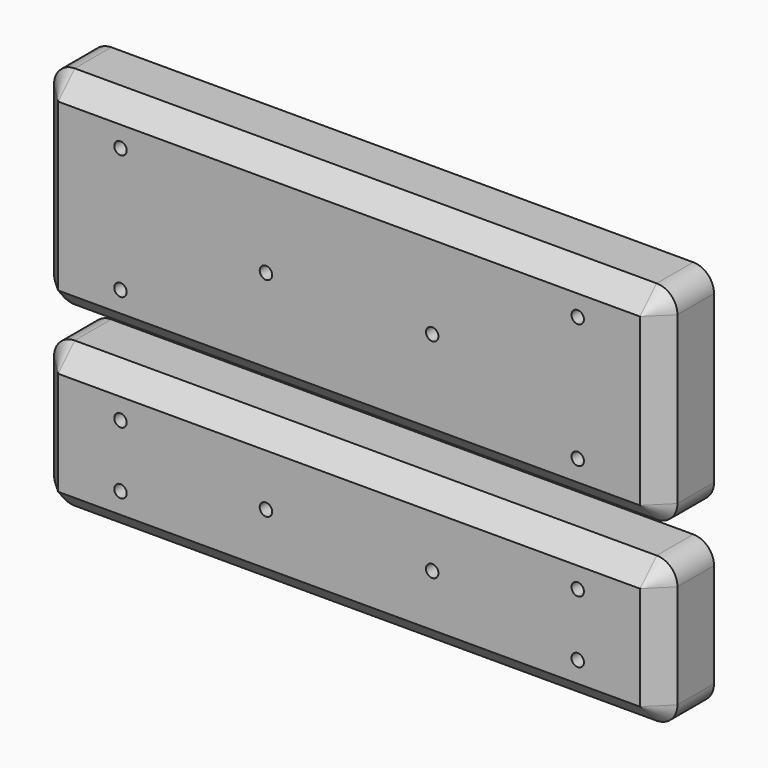
from build123d import *

# Parameters (mm, degrees)
F0_R      = 1.5
F1_DEPTH  = 16
F2_SIZE   = 4.99999
F2_2_SIZE = 4.99999


# Not quite as in the source:
# - a fillet or chamfer is up to 0.001 mm smaller than in the source, because OpenCascade refuses the exact size


with BuildPart() as f1:
    # F0 (on Front) → F1 (new body)
    with BuildSketch(Plane.XZ):
        with BuildLine():
            Line((70, 25), (-70, 25))
            ThreePointArc((-70, 25), (-73.5355339059, 23.5355339059), (-75, 20))
            Line((-75, 20), (-75, -20))
            ThreePointArc((-75, -20), (-73.5355339059, -23.5355339059), (-70, -25))
            Line((-70, -25), (70, -25))
            ThreePointArc((70, -25), (73.5355339059, -23.5355339059), (75, -20))
            Line((75, -20), (75, 20))
            ThreePointArc((75, 20), (73.5355339059, 23.5355339059), (70, 25))
        make_face()
        with Locations((-55, -15)):
            Circle(F0_R, mode=Mode.SUBTRACT)
        with Locations((-20, 0)):
            Circle(F0_R, mode=Mode.SUBTRACT)
        with Locations((-55, 15)):
            Circle(F0_R, mode=Mode.SUBTRACT)
        with Locations((20, 0)):
            Circle(F0_R, mode=Mode.SUBTRACT)
        with Locations((55, -15)):
            Circle(F0_R, mode=Mode.SUBTRACT)
        with Locations((55, 15)):
            Circle(F0_R, mode=Mode.SUBTRACT)
    extrude(amount=F1_DEPTH)

    # F2 (size 5 in the source; OpenCascade refuses exactly that, so slightly less here)
    f2_edges = [f1.edges().sort_by_distance(p)[0] for p in [
        (0, -16, 25),
        (-73.535534, -16, 23.535534),
        (-75, -16, 0),
        (-73.535534, -16, -23.535534),
        (0, -16, -25),
        (73.535534, -16, -23.535534),
        (75, -16, 0),
        (73.535534, -16, 23.535534),
    ]]
    chamfer(f2_edges, length=F2_SIZE)


with BuildPart() as f1b:
    # F0 (on Front) → F1, piece 2 (new body)
    with BuildSketch(Plane.XZ):
        with BuildLine():
            ThreePointArc((-70, -32.6368902624), (-73.5355339059, -34.1013563564), (-75, -37.6368902624))
            Line((-75, -37.6368902624), (-75, -62.6368902624))
            ThreePointArc((-75, -62.6368902624), (-73.5355339059, -66.1724241683), (-70, -67.6368902624))
            Line((-70, -67.6368902624), (70, -67.6368902624))
            ThreePointArc((70, -67.6368902624), (73.5355339059, -66.1724241683), (75, -62.6368902624))
            Line((75, -62.6368902624), (75, -37.6368902624))
            ThreePointArc((75, -37.6368902624), (73.5355339059, -34.1013563564), (70, -32.6368902624))
            Line((70, -32.6368902624), (-70, -32.6368902624))
        make_face()
        with Locations((-55, -57.6368902624)):
            Circle(F0_R, mode=Mode.SUBTRACT)
        with Locations((-20, -50.1368902624)):
            Circle(F0_R, mode=Mode.SUBTRACT)
        with Locations((-55, -42.6368902624)):
            Circle(F0_R, mode=Mode.SUBTRACT)
        with Locations((20, -50.1368902624)):
            Circle(F0_R, mode=Mode.SUBTRACT)
        with Locations((55, -57.6368902624)):
            Circle(F0_R, mode=Mode.SUBTRACT)
        with Locations((55, -42.6368902624)):
            Circle(F0_R, mode=Mode.SUBTRACT)
    extrude(amount=F1_DEPTH)

    # F2#2 (size 5 in the source; OpenCascade refuses exactly that, so slightly less here)
    f2_2_edges = [f1b.edges().sort_by_distance(p)[0] for p in [
        (0, -16, -32.63689),
        (0, -16, -67.63689),
        (73.535534, -16, -66.172424),
        (75, -16, -50.13689),
        (73.535534, -16, -34.101356),
        (-73.535534, -16, -34.101356),
        (-75, -16, -50.13689),
        (-73.535534, -16, -66.172424),
    ]]
    chamfer(f2_2_edges, length=F2_2_SIZE)


solid = Compound([f1.part, f1b.part])
